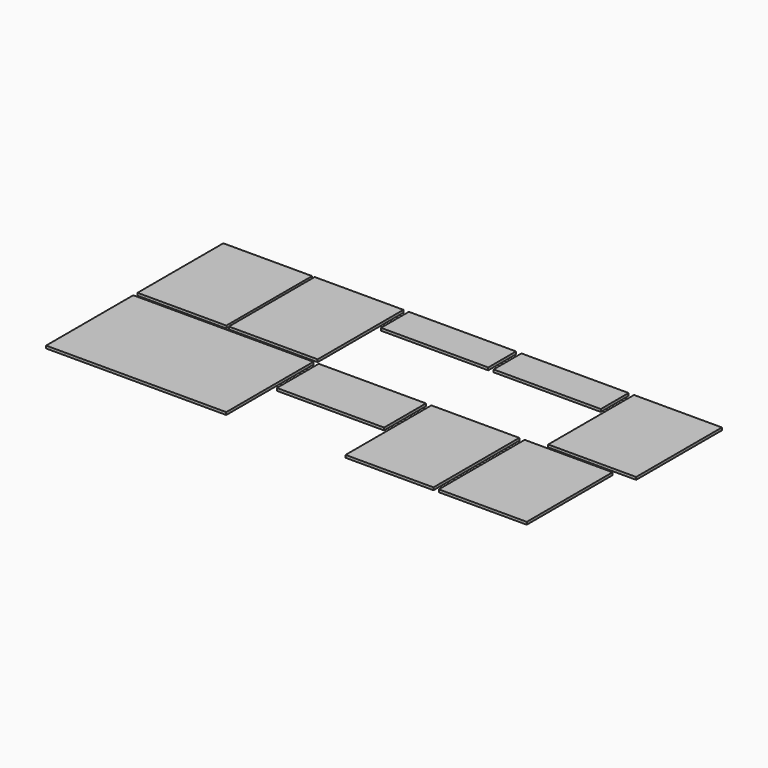
from build123d import *

# Parameters (mm, degrees)
F0_W     = 12
F0_H     = 500
F0_W_2   = 402
F1_DEPTH = 12
F0_W_3   = 840
F0_H_2   = 508
F0_W_4   = 500
F0_H_3   = 162
F0_H_4   = 244
F0_W_5   = 410


# Not quite as in the source:
# - a feature names something its author has since deleted; it is built from what else it names


with BuildPart() as f1:
    # F0 (on Top) → F1 (new body)
    with BuildSketch(Plane.XY):
        with Locations((-1340.6781625152, -61.1715600074)):
            Rectangle(F0_W, F0_H)
        with Locations((-1133.6781625152, -61.1715600074)):
            Rectangle(F0_W_2, F0_H)
    extrude(amount=F1_DEPTH)


with BuildPart() as f1b:
    # F0 (on Top) → F1, piece 2 (new body)
    with BuildSketch(Plane.XY):
        with Locations((-719.6781625152, -61.1715600074)):
            Rectangle(F0_W_2, F0_H)
        with Locations((-512.6781625152, -61.1715600074)):
            Rectangle(F0_W, F0_H)
    extrude(amount=F1_DEPTH)


with BuildPart() as f1c:
    # F0 (on Top) → F1, piece 3 (new body)
    with BuildSketch(Plane.XY):
        with Locations((-926.6781625152, -590.1715600074)):
            Rectangle(F0_W_3, F0_H_2)
    extrude(amount=F1_DEPTH)


with BuildPart() as f1d:
    # F0 (on Top) → F1, piece 4 (new body)
    with BuildSketch(Plane.XY):
        with Locations((-231.6781625152, 107.8284399926)):
            Rectangle(F0_W_4, F0_H_3)
    extrude(amount=F1_DEPTH)


with BuildPart() as f1e:
    # F0 (on Top) → F1, piece 5 (new body)
    with BuildSketch(Plane.XY):
        with Locations((-231.6781625152, -458.1715600074)):
            Rectangle(F0_W_4, F0_H_4)
    extrude(amount=F1_DEPTH)


with BuildPart() as f1f:
    # F0 (on Top) → F1, piece 6 (new body)
    with BuildSketch(Plane.XY):
        with Locations((248.3218374848, -586.1715600074)):
            Rectangle(F0_W_5, F0_H)
    extrude(amount=F1_DEPTH)


with BuildPart() as f1g:
    # F0 (on Top) → F1, piece 7 (new body)
    with BuildSketch(Plane.XY):
        with Locations((293.3218374848, 107.8284399926)):
            Rectangle(F0_W_4, F0_H_3)
    extrude(amount=F1_DEPTH)


with BuildPart() as f1h:
    # F0 (on Top) → F1, piece 8 (new body)
    with BuildSketch(Plane.XY):
        with Locations((683.3218374848, -586.1715600074)):
            Rectangle(F0_W_5, F0_H)
    extrude(amount=F1_DEPTH)


with BuildPart() as f1i:
    # F0 (on Top) → F1, piece 9 (new body)
    with BuildSketch(Plane.XY):
        with Locations((773.3218374848, -61.1715600074)):
            Rectangle(F0_W_5, F0_H)
    extrude(amount=F1_DEPTH)


solid = Compound([f1.part, f1b.part, f1c.part, f1d.part, f1e.part, f1f.part, f1g.part, f1h.part, f1i.part])
